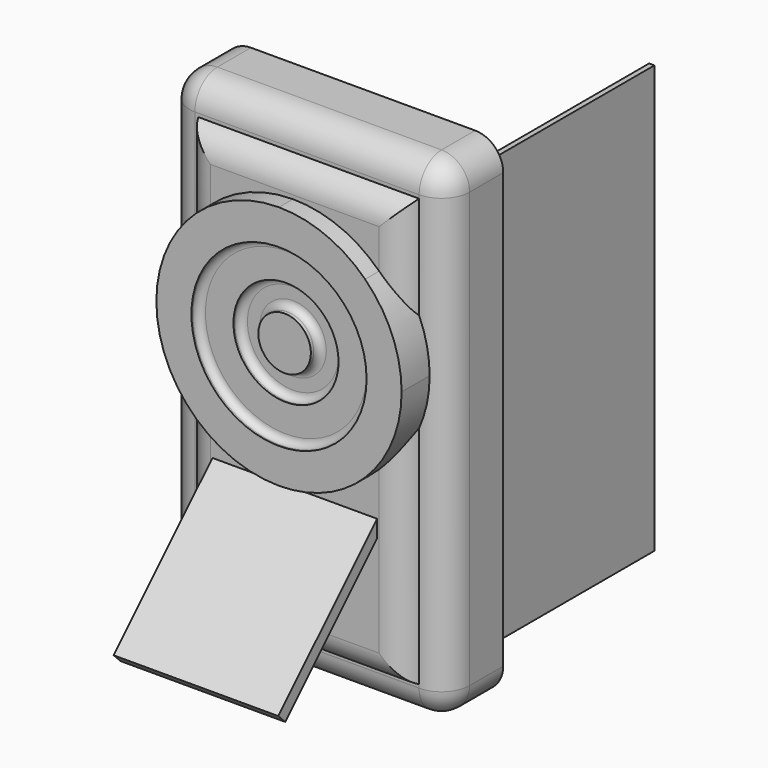
from build123d import *

# Parameters (mm, degrees)
F0_W         = 63
F0_H         = 122
F1_DEPTH     = 20
F2_DEPTH     = 25
F3_DEPTH     = 10
F4_T1_DEPTH  = 32
F4_T3_DEPTH  = 64
F4_T5_DEPTH  = 124
F4_T7_DEPTH  = 159.0809924355
F4_T9_DEPTH  = 100.0809924355
F4_S13_W     = 8.16
F4_S13_H     = 8.16
F4_T14_DEPTH = 8.16
F4_S19_W     = 8.16
F4_S19_H     = 8.16
F4_T20_DEPTH = 8.16
F4_S25_W     = 8.16
F4_S25_H     = 8.16
F4_T26_DEPTH = 8.16
F4_S31_W     = 8.16
F4_S31_H     = 8.16
F4_T32_DEPTH = 8.16
F5_W         = 1.5
F5_H         = 15
F6_DEPTH     = 1.5
F7_R         = 1.49999
F7_2_R       = 1.49999
F8_W         = 0.75
F8_H         = 122
F9_DEPTH     = 63
F10_W        = 63
F10_H        = 122
F11_DEPTH    = 0.75
F13_DEPTH    = 64
F14_DEPTH    = 17
F16_DEPTH    = 5
F17_R        = 25
F18_DEPTH    = 2.5
F19_R        = 15
F20_DEPTH    = 2.5
F21_R        = 7.5
F22_DEPTH    = 3
F23_R        = 2


# Not quite as in the source:
# - a fillet or chamfer that OpenCascade refuses, or shapes differently, is made with other operations: its cross-section is extruded or revolved along the edge and cut away or added
# - a fillet or chamfer is up to 0.001 mm smaller than in the source, because OpenCascade refuses the exact size


with BuildPart() as f1:
    # F0 (on Front) → F1 (new body)
    with BuildSketch(Plane.XZ):
        Polygon((0, 140), (0, 0), (9, 0), (80, 0), (80, 140), align=None)
        with Locations((40.5, 70)):
            Rectangle(F0_W, F0_H, mode=Mode.SUBTRACT)
    extrude(amount=F1_DEPTH)

    # F0 (on Front) → F2 (join)
    with BuildSketch(Plane.XZ):
        with Locations((40.5, 70)):
            Rectangle(F0_W, F0_H)
    extrude(amount=F2_DEPTH)

    # F0 (on Front) → F3 (cut)
    with BuildSketch(Plane.XZ):
        with Locations((40.5, 70)):
            Rectangle(F0_W, F0_H)
    extrude(amount=F3_DEPTH, mode=Mode.SUBTRACT)

    # F4: fillet of radius 8 on 12 edges, made by hand

    # F4_s2 → F4_t1 (cut)
    with BuildSketch(Plane.XZ.offset(-20)):
        with BuildLine():
            ThreePointArc((0, 8), (2.3431457505, 2.3431457505), (8, 0))
            Line((8, 0), (8, -0.16))
            Line((8, -0.16), (-0.16, -0.16))
            Line((-0.16, -0.16), (-0.16, 8))
            Line((-0.16, 8), (0, 8))
        make_face()
        with BuildLine():
            ThreePointArc((72, 0), (77.6568542495, 2.3431457505), (80, 8))
            Line((80, 8), (80.16, 8))
            Line((80.16, 8), (80.16, -0.16))
            Line((80.16, -0.16), (72, -0.16))
            Line((72, -0.16), (72, 0))
        make_face()
        with BuildLine():
            ThreePointArc((0, 132), (2.3431457505, 137.6568542495), (8, 140))
            Line((8, 140), (8, 140.16))
            Line((8, 140.16), (-0.16, 140.16))
            Line((-0.16, 140.16), (-0.16, 132))
            Line((-0.16, 132), (0, 132))
        make_face()
        with BuildLine():
            ThreePointArc((72, 140), (77.6568542495, 137.6568542495), (80, 132))
            Line((80, 132), (80.16, 132))
            Line((80.16, 132), (80.16, 140.16))
            Line((80.16, 140.16), (72, 140.16))
            Line((72, 140.16), (72, 140))
        make_face()
    extrude(amount=F4_T1_DEPTH, mode=Mode.SUBTRACT)

    # F4_s4 → F4_t3 (cut)
    with BuildSketch(Plane.YZ.offset(8)):
        with BuildLine():
            ThreePointArc((-12, 140), (-17.6568542495, 137.6568542495), (-20, 132))
            Line((-20, 132), (-20.16, 132))
            Line((-20.16, 132), (-20.16, 140.16))
            Line((-20.16, 140.16), (-12, 140.16))
            Line((-12, 140.16), (-12, 140))
        make_face()
        with BuildLine():
            ThreePointArc((-12, 0), (-17.6568542495, 2.3431457505), (-20, 8))
            Line((-20, 8), (-20.16, 8))
            Line((-20.16, 8), (-20.16, -0.16))
            Line((-20.16, -0.16), (-12, -0.16))
            Line((-12, -0.16), (-12, 0))
        make_face()
    extrude(amount=F4_T3_DEPTH, mode=Mode.SUBTRACT)

    # F4_s6 → F4_t5 (cut)
    with BuildSketch(Plane.XY.offset(8)):
        with BuildLine():
            ThreePointArc((0, -12), (2.3431457505, -17.6568542495), (8, -20))
            Line((8, -20), (8, -20.16))
            Line((8, -20.16), (-0.16, -20.16))
            Line((-0.16, -20.16), (-0.16, -12))
            Line((-0.16, -12), (0, -12))
        make_face()
        with BuildLine():
            ThreePointArc((72, -20), (77.6568542495, -17.6568542495), (80, -12))
            Line((80, -12), (80.16, -12))
            Line((80.16, -12), (80.16, -20.16))
            Line((80.16, -20.16), (72, -20.16))
            Line((72, -20.16), (72, -20))
        make_face()
    extrude(amount=F4_T5_DEPTH, mode=Mode.SUBTRACT)

    # F4_s8 → F4_t7 (cut)
    with BuildSketch(Plane.XY.offset(-9.5404962177)):
        with BuildLine():
            ThreePointArc((72, -20), (69.0559374679, -23.6332495807), (64.5838015129, -25))
            Line((64.5838015129, -25), (64.5838015129, -25.16))
            Line((64.5838015129, -25.16), (72, -25.16))
            Line((72, -25.16), (72.16, -25))
            ThreePointArc((72.16, -25), (72.16, -22.5), (72.1483239697, -20.06))
            Line((72.1483239697, -20.06), (72, -20))
        make_face()
        with BuildLine():
            ThreePointArc((9, -20), (11.9440625321, -23.6332495807), (16.4161984871, -25))
            Line((16.4161984871, -25), (16.4161984871, -25.16))
            Line((16.4161984871, -25.16), (9, -25.16))
            Line((9, -25.16), (8.84, -25))
            ThreePointArc((8.84, -25), (8.84, -22.5), (8.8516760303, -20.06))
            Line((8.8516760303, -20.06), (9, -20))
        make_face()
    extrude(amount=F4_T7_DEPTH, mode=Mode.SUBTRACT)

    # F4_s10 → F4_t9 (cut)
    with BuildSketch(Plane.YZ.offset(-9.5404962177)):
        with BuildLine():
            ThreePointArc((-20, 131), (-23.6332495807, 128.0559374679), (-25, 123.5838015129))
            Line((-25, 123.5838015129), (-25.16, 123.5838015129))
            Line((-25.16, 123.5838015129), (-25.16, 131))
            Line((-25.16, 131), (-25, 131.16))
            ThreePointArc((-25, 131.16), (-22.5, 131.16), (-20.06, 131.1483239697))
            Line((-20.06, 131.1483239697), (-20, 131))
        make_face()
        with BuildLine():
            ThreePointArc((-20, 9), (-23.6332495807, 11.9440625321), (-25, 16.4161984871))
            Line((-25, 16.4161984871), (-25.16, 16.4161984871))
            Line((-25.16, 16.4161984871), (-25.16, 9))
            Line((-25.16, 9), (-25, 8.84))
            ThreePointArc((-25, 8.84), (-22.5, 8.84), (-20.06, 8.8516760303))
            Line((-20.06, 8.8516760303), (-20, 9))
        make_face()
    extrude(amount=F4_T9_DEPTH, mode=Mode.SUBTRACT)


with BuildPart() as f4_tool12:
    # F4_s13 → F4_t14 (new body)
    with BuildSketch(Plane.YZ.offset(8)):
        with Locations((-16.08, 3.92)):
            Rectangle(F4_S13_W, F4_S13_H)
    extrude(amount=-F4_T14_DEPTH)

    # F4_s15 → F4_t16 (revolve, cut)
    with BuildSketch(Plane(origin=(8, -12, 8), x_dir=(0, 0.7071067812, 0.7071067812), z_dir=(0, -0.7071067812, 0.7071067812))):
        with BuildLine():
            ThreePointArc((0, -8), (8, 0), (0, 8))
            Line((0, 8), (0, -8))
        make_face()
    revolve(axis=Axis((8, -12, 8), (-1, 0, 0)), mode=Mode.SUBTRACT)


with BuildPart() as f1_1:
    add(f1.part)

    # F4_t11: cut F4_tool12
    add(f4_tool12.part, mode=Mode.SUBTRACT)


with BuildPart() as f4_tool18:
    # F4_s19 → F4_t20 (new body)
    with BuildSketch(Plane.XY.offset(8)):
        with Locations((76.08, -16.08)):
            Rectangle(F4_S19_W, F4_S19_H)
    extrude(amount=-F4_T20_DEPTH)

    # F4_s21 → F4_t22 (revolve, cut)
    with BuildSketch(Plane(origin=(72, -12, 8), x_dir=(-0.7071067812, 0.7071067812, 0), z_dir=(-0.7071067812, -0.7071067812, 0))):
        with BuildLine():
            ThreePointArc((0, -8), (8, 0), (0, 8))
            Line((0, 8), (0, -8))
        make_face()
    revolve(axis=Axis((72, -12, 8), (0, 0, -1)), mode=Mode.SUBTRACT)


with BuildPart() as f1_2:
    add(f1_1.part)

    # F4_t17: cut F4_tool18
    add(f4_tool18.part, mode=Mode.SUBTRACT)


with BuildPart() as f4_tool24:
    # F4_s25 → F4_t26 (new body)
    with BuildSketch(Plane.YZ.offset(8)):
        with Locations((-16.08, 136.08)):
            Rectangle(F4_S25_W, F4_S25_H)
    extrude(amount=-F4_T26_DEPTH)

    # F4_s27 → F4_t28 (revolve, cut)
    with BuildSketch(Plane(origin=(8, -12, 132), x_dir=(0, 0.7071067812, -0.7071067812), z_dir=(0, 0.7071067812, 0.7071067812))):
        with BuildLine():
            ThreePointArc((0, -8), (8, 0), (0, 8))
            Line((0, 8), (0, -8))
        make_face()
    revolve(axis=Axis((8, -12, 132), (-1, 0, 0)), mode=Mode.SUBTRACT)


with BuildPart() as f1_3:
    add(f1_2.part)

    # F4_t23: cut F4_tool24
    add(f4_tool24.part, mode=Mode.SUBTRACT)


with BuildPart() as f4_tool30:
    # F4_s31 → F4_t32 (new body)
    with BuildSketch(Plane.XY.offset(132)):
        with Locations((76.08, -16.08)):
            Rectangle(F4_S31_W, F4_S31_H)
    extrude(amount=F4_T32_DEPTH)

    # F4_s33 → F4_t34 (revolve, cut)
    with BuildSketch(Plane(origin=(72, -12, 132), x_dir=(-0.7071067812, 0.7071067812, 0), z_dir=(0.7071067812, 0.7071067812, 0))):
        with BuildLine():
            ThreePointArc((0, -8), (8, 0), (0, 8))
            Line((0, 8), (0, -8))
        make_face()
    revolve(axis=Axis((72, -12, 132), (0, 0, 1)), mode=Mode.SUBTRACT)


with BuildPart() as f1_4:
    add(f1_3.part)

    # F4_t29: cut F4_tool30
    add(f4_tool30.part, mode=Mode.SUBTRACT)

    # F12 (on Right) → F13 (join)
    with BuildSketch(Plane.YZ):
        Polygon((-57.7781745931, 12.2720779386), (-25, 45.0502525317), (-25, 50), (-50, 25), (-60.2530483272, 14.7469516728), align=None)
    extrude(amount=F13_DEPTH)

    # F14 (cut): a face of the model
    f14_faces = [f1_4.faces().sort_by_distance(p)[0] for p in [
        (0, -42.0153084126, 30.5398285833),
    ]]
    extrude(f14_faces, amount=-F14_DEPTH, mode=Mode.SUBTRACT)

    # F15 (on face) → F16 (join, symmetric)
    with BuildSketch(Plane.XZ.offset(25)):
        with BuildLine():
            Line((40, 52.5), (40, 70))
            Line((40, 70), (40, 87.5))
            Line((40, 87.5), (40, 105))
            Line((40, 105), (40, 122.5))
            ThreePointArc((40, 122.5), (27.3537315182, 120.1354392262), (16.4161984871, 113.3612510564))
            Line((16.4161984871, 113.3612510564), (16.4161984871, 61.6387489436))
            ThreePointArc((16.4161984871, 61.6387489436), (27.3537315182, 54.8645607738), (40, 52.5))
        make_face()
        with BuildLine():
            Line((40, 87.5), (40, 70))
            Line((40, 70), (40, 52.5))
            ThreePointArc((40, 52.5), (53.2864528225, 55.1199108804), (64.5838015129, 62.5874187774))
            Line((64.5838015129, 62.5874187774), (64.5838015129, 112.4125812226))
            ThreePointArc((64.5838015129, 112.4125812226), (53.2864528225, 119.8800891196), (40, 122.5))
            Line((40, 122.5), (40, 105))
            Line((40, 105), (40, 87.5))
        make_face()
        with BuildLine():
            ThreePointArc((16.4161984871, 113.3612510564), (5, 87.5), (16.4161984871, 61.6387489436))
            Line((16.4161984871, 61.6387489436), (16.4161984871, 113.3612510564))
        make_face()
        with BuildLine():
            Line((64.5838015129, 112.4125812226), (64.5838015129, 62.5874187774))
            ThreePointArc((64.5838015129, 62.5874187774), (72.2911214806, 73.9987602968), (75, 87.5))
            ThreePointArc((75, 87.5), (72.2911214806, 101.0012397032), (64.5838015129, 112.4125812226))
        make_face()
    extrude(amount=F16_DEPTH, both=True)

    # F17 (on face) → F18 (cut)
    with BuildSketch(Plane.XZ.offset(30)):
        with Locations((40, 87.5)):
            Circle(F17_R)
    extrude(amount=-F18_DEPTH, mode=Mode.SUBTRACT)

    # F19 (on face) → F20 (cut)
    with BuildSketch(Plane.XZ.offset(27.5)):
        with Locations((40, 87.5)):
            Circle(F19_R)
    extrude(amount=-F20_DEPTH, mode=Mode.SUBTRACT)

    # F21 (on face) → F22 (join)
    with BuildSketch(Plane.XZ.offset(25)):
        with Locations((40, 87.5)):
            Circle(F21_R)
    extrude(amount=F22_DEPTH)

    # F23
    f23_edges = [f1_4.edges().sort_by_distance(p)[0] for p in [
        (15, -27.5, 87.5),
        (25, -25, 87.5),
        (32.5, -25, 87.5),
    ]]
    fillet(f23_edges, radius=F23_R)


with BuildPart() as f6:
    # F5 (on face) → F6 (new body, symmetric)
    with BuildSketch(Plane.XZ):
        with Locations((72.75, 105.75)):
            Rectangle(F5_W, F5_H)
        with Locations((71.25, 105.75)):
            Rectangle(F5_W, F5_H)
    extrude(amount=F6_DEPTH, both=True)

    # F7 (radius 1.5 in the source; OpenCascade refuses exactly that, so slightly less here)
    f7_edges = [f6.edges().sort_by_distance(p)[0] for p in [
        (73.5, 1.5, 105.75),
        (70.5, 1.5, 105.75),
        (70.5, -1.5, 105.75),
    ]]
    fillet(f7_edges, radius=F7_R)


with BuildPart() as f6b:
    # F5 (on face) → F6, piece 2 (new body, symmetric)
    with BuildSketch(Plane.XZ):
        with Locations((72.75, 25.25)):
            Rectangle(F5_W, F5_H)
        with Locations((71.25, 25.25)):
            Rectangle(F5_W, F5_H)
    extrude(amount=F6_DEPTH, both=True)

    # F7#2 (radius 1.5 in the source; OpenCascade refuses exactly that, so slightly less here)
    f7_2_edges = [f6b.edges().sort_by_distance(p)[0] for p in [
        (73.5, 1.5, 25.25),
        (70.5, 1.5, 25.25),
        (70.5, -1.5, 25.25),
    ]]
    fillet(f7_2_edges, radius=F7_2_R)


with BuildPart() as f9:
    # F8 (on Front) → F9 (new body)
    with BuildSketch(Plane.XZ):
        with Locations((71.625, 70)):
            Rectangle(F8_W, F8_H)
        with Locations((72.375, 70)):
            Rectangle(F8_W, F8_H)
    extrude(amount=-F9_DEPTH)


with BuildPart() as f11:
    # F10 (on Front) → F11 (new body, symmetric)
    with BuildSketch(Plane.XZ):
        with Locations((40.5, 70)):
            Rectangle(F10_W, F10_H)
    extrude(amount=F11_DEPTH, both=True)


solid = Compound([f1_4.part, f6.part, f6b.part, f9.part, f11.part])
